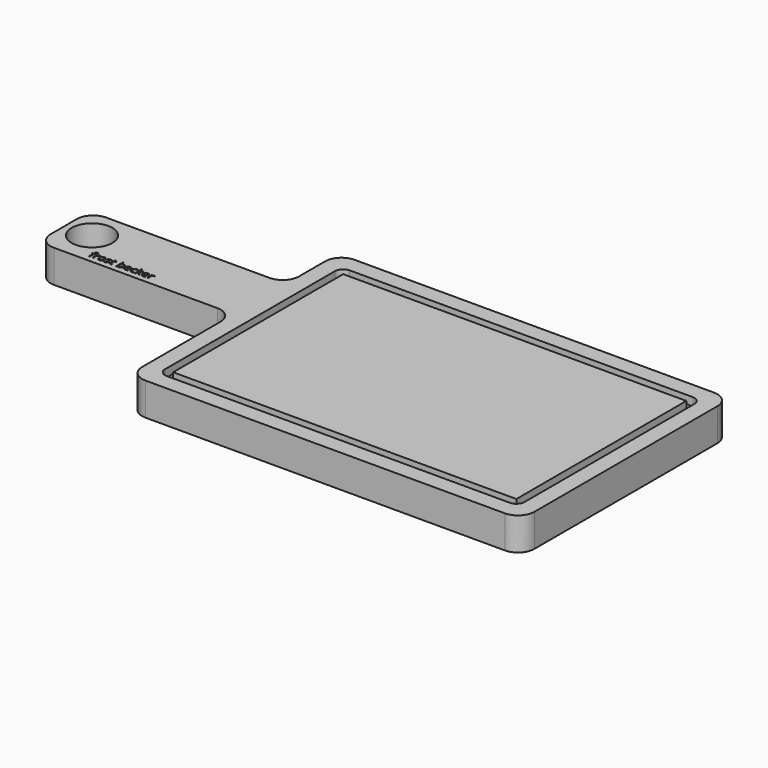
from build123d import *

# Parameters (mm, degrees)
F0_W         = 152.4
F0_H         = 50.8
F1_DEPTH     = 25.4
F2_R         = 15.875
F3_DEPTH     = 25.4
F4_DEPTH     = 6.35
F5_R         = 6.35
F6_R         = 12.7
F7_TEXT_SIZE = 8.7802608808
F8_DEPTH     = 2.54


# Not quite as in the source:
# - Text() gives the source's letters only with a copy of the font that has no kerning and outlines rounded to 1/6400 em; it was checked with that copy


with BuildPart() as f1:
    # F0 (on Top) → F1 (new body)
    with BuildSketch(Plane.XY):
        with Locations((-76.2, 127)):
            Rectangle(F0_W, F0_H)
        Polygon((0, 101.6), (0, 0), (304.8, 0), (304.8, 203.2), (0, 203.2), (0, 152.4), align=None)
    extrude(amount=F1_DEPTH)

    # F2 (on face) → F3 (cut)
    with BuildSketch(Plane.XY.offset(25.4)):
        with Locations((-131.7903697491, 128.7244409323)):
            Circle(F2_R)
    extrude(amount=-F3_DEPTH, mode=Mode.SUBTRACT)

    # F2 (on face) → F4 (cut)
    with BuildSketch(Plane.XY.offset(25.4)):
        with Locations((-131.7903697491, 128.7244409323)):
            Circle(F2_R)
        Polygon((12.6999939203, 101.6), (12.6999939203, 12.6999939203), (292.1000060797, 12.6999939203), (292.1000060797, 190.5000060797), (12.6999939203, 190.5000060797), (12.6999939203, 152.4), align=None)
        Polygon((19.0499939203, 101.6), (19.0499939203, 152.4), (19.0499939203, 184.1500060797), (285.7500060797, 184.1500060797), (285.7500060797, 19.0499939203), (19.0499939203, 19.0499939203), align=None, mode=Mode.SUBTRACT)
    extrude(amount=-F4_DEPTH, mode=Mode.SUBTRACT)

    # F5
    f5_edges = [f1.edges().sort_by_distance(p)[0] for p in [
        (12.699994, 190.500006, 22.225),
        (12.699994, 12.699994, 22.225),
        (292.100006, 190.500006, 22.225),
        (292.100006, 12.699994, 22.225),
    ]]
    fillet(f5_edges, radius=F5_R)

    # F6
    f6_edges = [f1.edges().sort_by_distance(p)[0] for p in [
        (0, 203.2, 12.7),
        (0, 0, 12.7),
        (-152.4, 152.4, 12.7),
        (-152.4, 101.6, 12.7),
        (304.8, 0, 12.7),
        (304.8, 203.2, 12.7),
        (0, 152.4, 12.7),
        (0, 101.6, 12.7),
    ]]
    fillet(f6_edges, radius=F6_R)

    # F7 (on face) → F8 (cut)
    with BuildSketch(Plane.XY.offset(25.4)):
        with Locations((-117.1850264072, 106.1872020364)):
            Text('frost becker', F7_TEXT_SIZE, font='Open Sans', text_align=(TextAlign.LEFT, TextAlign.BOTTOM))
    extrude(amount=-F8_DEPTH, mode=Mode.SUBTRACT)


solid = f1.part
